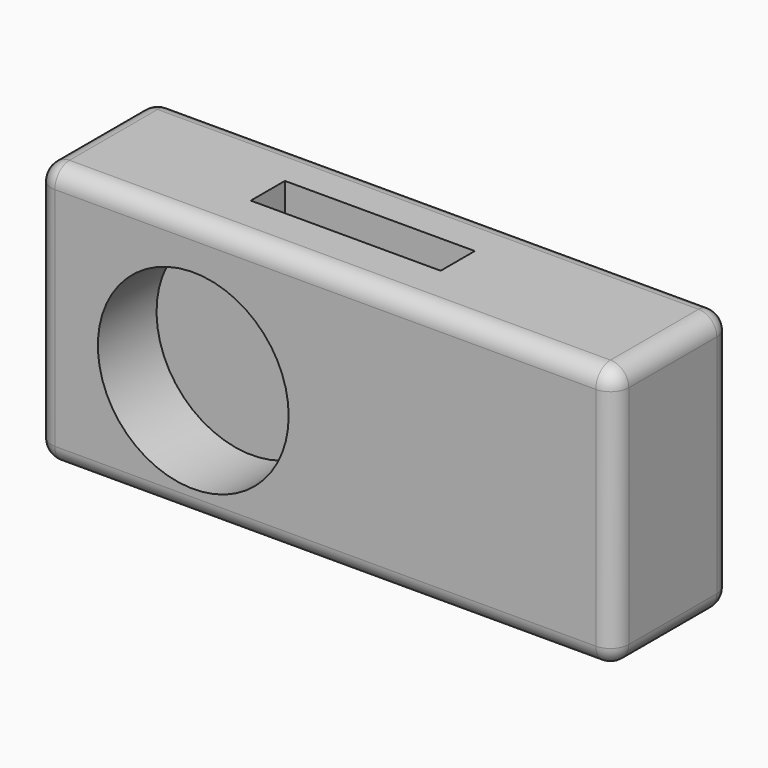
from build123d import *

# Parameters (mm, degrees)
F0_W     = 157.5113609433
F0_H     = 71.6332271695
F1_DEPTH = 40
F2_R     = 5
F3_R     = 26.0186453027
F4_DEPTH = 20
F5_W     = 51.7887976021
F5_H     = 11.637929827
F6_DEPTH = 35
F7_R     = 5


# Not quite as in the source:
# - the program builds the solid bodies; features that only make, move or delete a surface that nothing else refers to are left out


with BuildPart() as f1:
    # F0 (on Front) → F1 (new body)
    with BuildSketch(Plane.XZ):
        with Locations((3.7253e-06, 35.8166135848)):
            Rectangle(F0_W, F0_H)
    extrude(amount=F1_DEPTH)

    # F2
    f2_edges = [f1.edges().sort_by_distance(p)[0] for p in [
        (4e-06, -40, 71.633227),
        (4e-06, 0, 71.633227),
        (78.755684, -40, 35.816614),
        (78.755684, 0, 35.816614),
        (78.755684, -20, 71.633227),
        (-78.755677, -20, 71.633227),
        (-78.755677, 0, 35.816614),
        (-78.755677, -40, 35.816614),
    ]]
    fillet(f2_edges, radius=F2_R)

    # F3 (on face) → F4 (cut)
    with BuildSketch(Plane.XZ.offset(40)):
        with Locations((-36.0129252076, 33.036891371)):
            Circle(F3_R)
    extrude(amount=-F4_DEPTH, mode=Mode.SUBTRACT)

    # F5 (on face) → F6 (cut)
    with BuildSketch(Plane.XY.offset(71.6332271695)):
        with Locations((-6.1099091545, -19.590517506)):
            Rectangle(F5_W, F5_H)
    extrude(amount=-F6_DEPTH, mode=Mode.SUBTRACT)

    # F7
    f7_edges = [f1.edges().sort_by_distance(p)[0] for p in [
        (4e-06, -40, 0),
    ]]
    fillet(f7_edges, radius=F7_R)


solid = f1.part
